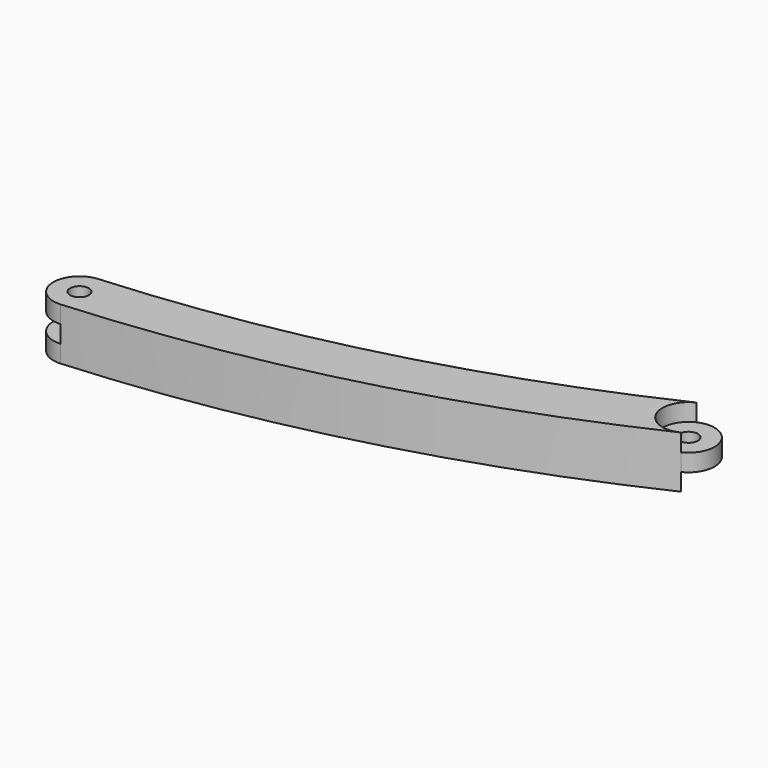
from build123d import *

# Parameters (mm, degrees)
F1_DEPTH = 15
F0_R     = 2.7
F2_DEPTH = 5
F3_START = 10
F3_DEPTH = 5
F4_START = 5
F4_DEPTH = 5


with BuildPart() as f1:
    # F0 (on Top) → F1 (new body)
    with BuildSketch(Plane.XY):
        with BuildLine():
            ThreePointArc((128.9690721838, 41.7179030249), (59.4297181842, 16.601757413), (-13.5443023154, 4.7133236555))
            ThreePointArc((-13.5443023154, 4.7133236555), (-5.5454612916, -2.2522016138), (-12.5109865609, -10.2510426376))
            ThreePointArc((-12.5109865609, -10.2510426376), (63.1995597074, 2.0832073859), (135.346639482, 28.1412084582))
            ThreePointArc((135.346639482, 28.1412084582), (125.3695085496, 31.7407720924), (128.9690721838, 41.7179030249))
        make_face()
    extrude(amount=F1_DEPTH)

    # F0 (on Top) → F2 (join)
    with BuildSketch(Plane.XY):
        with BuildLine():
            ThreePointArc((-12.5109865609, -10.2510426376), (-5.5454612916, -2.2522016138), (-13.5443023154, 4.7133236555))
            ThreePointArc((-13.5443023154, 4.7133236555), (-20.5098275846, -3.2855173683), (-12.5109865609, -10.2510426376))
        make_face()
        with Locations((-13.0276444381, -2.768859491)):
            Circle(F0_R, mode=Mode.SUBTRACT)
    extrude(amount=F2_DEPTH)

    # F0 (on Top) → F3 (join)
    with BuildSketch(Plane.XY.offset(F3_START)):
        with BuildLine():
            ThreePointArc((-12.5109865609, -10.2510426376), (-5.5454612916, -2.2522016138), (-13.5443023154, 4.7133236555))
            ThreePointArc((-13.5443023154, 4.7133236555), (-20.5098275846, -3.2855173683), (-12.5109865609, -10.2510426376))
        make_face()
        with Locations((-13.0276444381, -2.768859491)):
            Circle(F0_R, mode=Mode.SUBTRACT)
    extrude(amount=F3_DEPTH)

    # F0 (on Top) → F4 (join)
    with BuildSketch(Plane.XY.offset(F4_START)):
        with BuildLine():
            ThreePointArc((135.346639482, 28.1412084582), (138.9462031162, 38.1183393907), (128.9690721838, 41.7179030249))
            ThreePointArc((128.9690721838, 41.7179030249), (125.3695085496, 31.7407720924), (135.346639482, 28.1412084582))
        make_face()
        with Locations((132.1578558329, 34.9295557416)):
            Circle(F0_R, mode=Mode.SUBTRACT)
    extrude(amount=F4_DEPTH)


solid = f1.part
